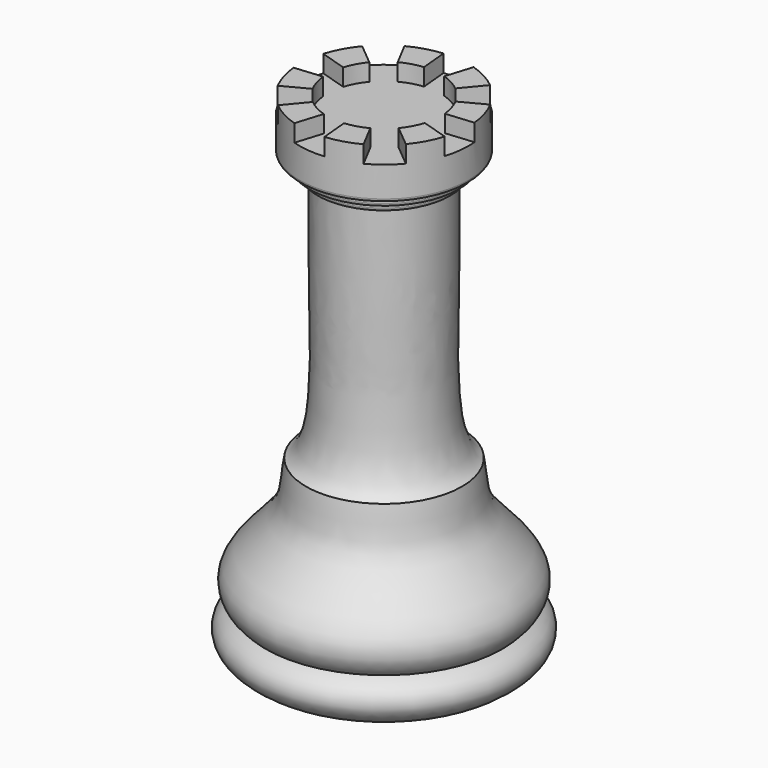
from build123d import *

# Parameters (mm, degrees)
F4_DEPTH = 4
F5_R     = 0.4


with BuildPart() as f1:
    # F0 (on Front) → F1 (revolve)
    with BuildSketch(Plane.XZ):
        with BuildLine():
            Line((7.4700926862, 14.109692609), (7.4700926862, -35.890307391))
            Line((7.4700926862, -35.890307391), (21.4700926862, -35.890307391))
            add(Edge.make_bspline(
                [(21.4700926862, -35.890307391), (22.9308548616, -35.015944948), (23.8569471054, -33.3210956528), (22.8896205888, -31.6196046119), (21.4700926862, -31.0222748667)],
                knots=[0, 0, 0, 0, 0.5110689786, 1, 1, 1, 1], degree=3))
            add(Edge.make_bspline(
                [(21.4700926862, -31.0222748667), (22.3144681852, -30.3379701873), (24.2188639082, -26.9328023049), (16.5762578768, -21.2234513875), (17.1360278665, -18.0033264541), (16.6927366865, -15.6595999994)],
                knots=[0, 0, 0, 0, 0.271010464, 0.6675538828, 1, 1, 1, 1], degree=3))
            add(Edge.make_bspline(
                [(14.4700926862, 14.109692609), (14.4700926862, -2.9557740159), (14.0108114789, -5.5993047887), (14.9732734996, -14.7046454667), (16.6927366865, -15.6595999994)],
                knots=[0, 0, 0, 0, 0.6460817935, 1, 1, 1, 1], degree=3))
            Line((14.4700926862, 14.109692609), (15.4700926862, 14.109692609))
            Line((15.4700926862, 14.109692609), (15.4700926862, 15.109692609))
            Line((15.4700926862, 15.109692609), (16.4700926862, 15.109692609))
            Line((16.4700926862, 15.109692609), (16.4700926862, 16.109692609))
            Line((16.4700926862, 16.109692609), (17.4700926862, 16.109692609))
            Line((17.4700926862, 16.109692609), (17.4700926862, 22.109692609))
            Line((17.4700926862, 22.109692609), (7.4700926862, 22.109692609))
            Line((7.4700926862, 22.109692609), (7.4700926862, 14.109692609))
        make_face()
    revolve(axis=Axis((7.4700926862, 0, -10.890307391), (0, 0, -1)))

    # F3 (on offset) → F4 (cut)
    with BuildSketch(Plane.XY.offset(24.07653)):
        with BuildLine():
            Line((-0.2219189679, 6.3900670351), (2.2999553212, 4.2950434592))
            ThreePointArc((2.2999553212, 4.2950434592), (1.5613766494, 3.20387164), (1.0498666213, 1.9895768305))
            Line((1.0498666213, 1.9895768305), (-2.0817722309, 2.9600467235))
            ThreePointArc((-2.0817722309, 2.9600467235), (-2.4757122934, 1.0396938532), (-2.4874406482, -0.9206138689))
            Line((-2.4874406482, -0.9206138689), (0.7771991403, -0.618784835))
            ThreePointArc((0.7771991403, -0.618784835), (1.0265201458, -1.912613815), (1.5234640304, -3.1329421187))
            Line((1.5234640304, -3.1329421187), (-1.3771648805, -4.6611193451))
            ThreePointArc((-1.3771648805, -4.6611193451), (-0.2978280332, -6.2975715715), (1.0800256511, -7.6920116541))
            Line((1.0800256511, -7.6920116541), (3.175049227, -5.170137365))
            ThreePointArc((3.175049227, -5.170137365), (4.2662210462, -5.9087160368), (5.4805158557, -6.4202260649))
            Line((5.4805158557, -6.4202260649), (4.5100459627, -9.5518649171))
            ThreePointArc((4.5100459627, -9.5518649171), (6.430398833, -9.9458049796), (8.390706555, -9.9575333343))
            Line((8.390706555, -9.9575333343), (8.0888775212, -6.6928935459))
            ThreePointArc((8.0888775212, -6.6928935459), (9.3827065012, -6.4435725404), (10.6030348049, -5.9466286558))
            Line((10.6030348049, -5.9466286558), (12.1312120312, -8.8472575667))
            ThreePointArc((12.1312120312, -8.8472575667), (13.7676642577, -7.7679207194), (15.1621043403, -6.3900670351))
            Line((15.1621043403, -6.3900670351), (12.6402300512, -4.2950434592))
            ThreePointArc((12.6402300512, -4.2950434592), (13.3788087229, -3.20387164), (13.8903187511, -1.9895768305))
            Line((13.8903187511, -1.9895768305), (17.0219576033, -2.9600467235))
            ThreePointArc((17.0219576033, -2.9600467235), (17.4158976658, -1.0396938532), (17.4276260205, 0.9206138689))
            Line((17.4276260205, 0.9206138689), (14.1629862321, 0.618784835))
            ThreePointArc((14.1629862321, 0.618784835), (13.9136652266, 1.912613815), (13.416721342, 3.1329421187))
            Line((13.416721342, 3.1329421187), (16.3173502529, 4.6611193451))
            ThreePointArc((16.3173502529, 4.6611193451), (15.2380134055, 6.2975715715), (13.8601597213, 7.6920116541))
            Line((13.8601597213, 7.6920116541), (11.7651361453, 5.170137365))
            ThreePointArc((11.7651361453, 5.170137365), (10.6739643262, 5.9087160368), (9.4596695167, 6.4202260649))
            Line((9.4596695167, 6.4202260649), (10.4301394097, 9.5518649171))
            ThreePointArc((10.4301394097, 9.5518649171), (8.5097865394, 9.9458049796), (6.5494788173, 9.9575333343))
            Line((6.5494788173, 9.9575333343), (6.8513078512, 6.6928935459))
            ThreePointArc((6.8513078512, 6.6928935459), (5.5574788712, 6.4435725404), (4.3371505675, 5.9466286558))
            Line((4.3371505675, 5.9466286558), (2.8089733411, 8.8472575667))
            ThreePointArc((2.8089733411, 8.8472575667), (1.1725211147, 7.7679207194), (-0.2219189679, 6.3900670351))
        make_face()
    extrude(amount=-F4_DEPTH, mode=Mode.SUBTRACT)

    # F5
    f5_edges = [f1.edges().sort_by_distance(p)[0] for p in [
        (-1.529907, 0, 15.109693),
        (-0.529907, 0, 14.109693),
        (-1.529907, 0, 16.109693),
        (-2.529907, 0, 16.109693),
    ]]
    fillet(f5_edges, radius=F5_R)


solid = f1.part
